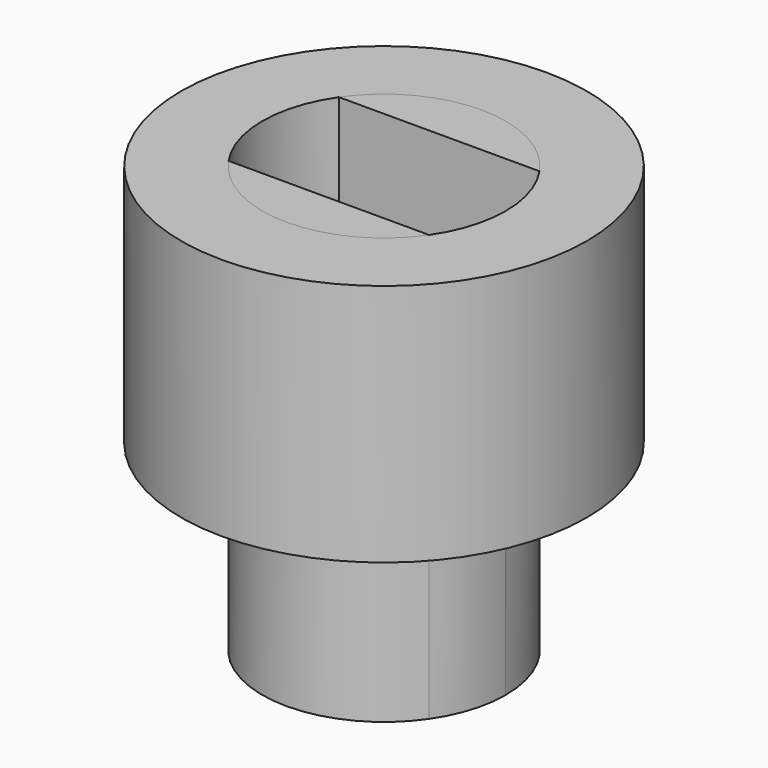
from build123d import *

# Parameters (mm, degrees)
F1_DEPTH = 4.5
F0_R     = 5
F2_DEPTH = 6
F3_DEPTH = 6
F4_DEPTH = 6


with BuildPart() as f1:
    # F0 (on Top) → F1 (new body)
    with BuildSketch(Plane.XY):
        with BuildLine():
            Line((1.7, 1.7), (2.4718414189, 1.7))
            ThreePointArc((2.4718414189, 1.7), (0, 3), (-2.4718414189, 1.7))
            Line((-2.4718414189, 1.7), (-1.7, 1.7))
            Line((-1.7, 1.7), (1.7, 1.7))
        make_face()
        with BuildLine():
            Line((-1.7, 1.7), (-2.4718414189, 1.7))
            ThreePointArc((-2.4718414189, 1.7), (-3, 0), (-2.4718414189, -1.7))
            Line((-2.4718414189, -1.7), (-1.7, -1.7))
            Line((-1.7, -1.7), (-1.7, 1.7))
        make_face()
        with BuildLine():
            ThreePointArc((-2.4718414189, -1.7), (0, -3), (2.4718414189, -1.7))
            Line((2.4718414189, -1.7), (1.7, -1.7))
            Line((1.7, -1.7), (-1.7, -1.7))
            Line((-1.7, -1.7), (-2.4718414189, -1.7))
        make_face()
        with BuildLine():
            ThreePointArc((2.4718414189, -1.7), (2.8649192185, -0.8900774526), (3, 0))
            ThreePointArc((3, 0), (2.8649192185, 0.8900774526), (2.4718414189, 1.7))
            Line((2.4718414189, 1.7), (1.7, 1.7))
            Line((1.7, 1.7), (1.7, -1.7))
            Line((1.7, -1.7), (2.4718414189, -1.7))
        make_face()
    extrude(amount=-F1_DEPTH)


with BuildPart() as f2:
    # F0 (on Top) → F2 (new body)
    with BuildSketch(Plane.XY):
        Circle(F0_R)
        with BuildLine():
            ThreePointArc((2.4718414189, 1.7), (2.8649192185, 0.8900774526), (3, 0))
            ThreePointArc((3, 0), (2.8649192185, -0.8900774526), (2.4718414189, -1.7))
            ThreePointArc((2.4718414189, -1.7), (0, -3), (-2.4718414189, -1.7))
            ThreePointArc((-2.4718414189, -1.7), (-3, 0), (-2.4718414189, 1.7))
            ThreePointArc((-2.4718414189, 1.7), (0, 3), (2.4718414189, 1.7))
        make_face(mode=Mode.SUBTRACT)
    extrude(amount=F2_DEPTH)


with BuildPart() as f3:
    # F0 (on Top) → F3 (new body)
    with BuildSketch(Plane.XY):
        with BuildLine():
            Line((1.7, 1.7), (2.4718414189, 1.7))
            ThreePointArc((2.4718414189, 1.7), (0, 3), (-2.4718414189, 1.7))
            Line((-2.4718414189, 1.7), (-1.7, 1.7))
            Line((-1.7, 1.7), (1.7, 1.7))
        make_face()
    extrude(amount=F3_DEPTH)


with BuildPart() as f4:
    # F0 (on Top) → F4 (new body)
    with BuildSketch(Plane.XY):
        with BuildLine():
            ThreePointArc((-2.4718414189, -1.7), (0, -3), (2.4718414189, -1.7))
            Line((2.4718414189, -1.7), (1.7, -1.7))
            Line((1.7, -1.7), (-1.7, -1.7))
            Line((-1.7, -1.7), (-2.4718414189, -1.7))
        make_face()
    extrude(amount=F4_DEPTH)


solid = Compound([f1.part, f2.part, f3.part, f4.part])
